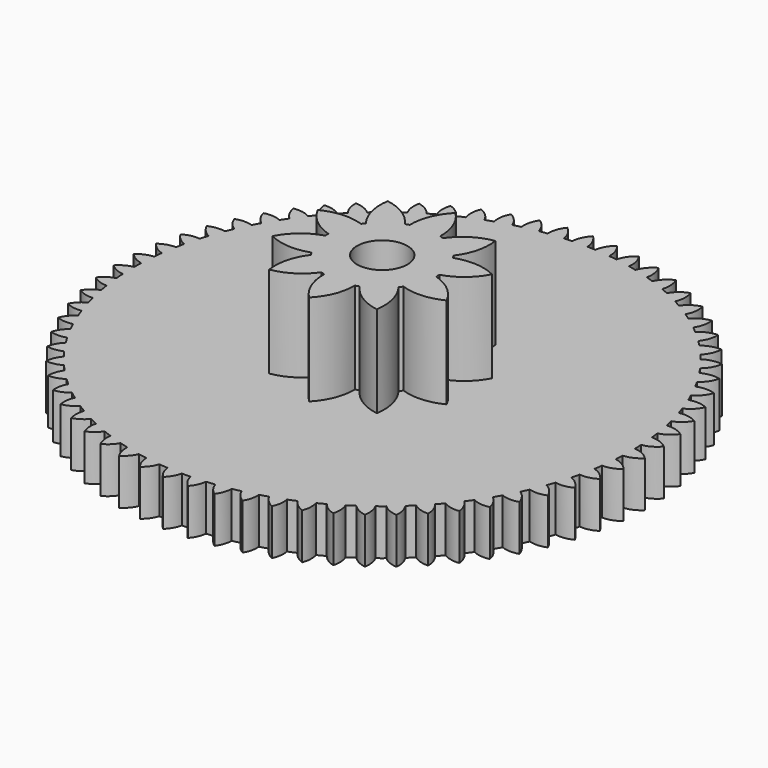
from build123d import *

# Parameters (mm, degrees)
F0_R     = 1.65
F1_DEPTH = 3
F2_R     = 1.65
F3_DEPTH = 6


# Not quite as in the source:
# - ends of sketch curves that miss each other by under 0.0002 mm in the source are joined


with BuildPart() as f1:
    # F0 (on Top) → F1 (new body)
    with BuildSketch(Plane.XY):
        with BuildLine():
            ThreePointArc((9.0030000822, 13.5880826286), (9.1966564399, 14.1755106046), (9.1611494678, 14.7930166101))
            ThreePointArc((9.1611494678, 14.7930166101), (8.5914009501, 14.5506518569), (8.1505703153, 14.1158847946))
            ThreePointArc((8.1505703153, 14.1158847946), (8.5808442549, 13.8585393124), (9.0030000822, 13.5880826286))
        make_face()
        with BuildLine():
            ThreePointArc((9.4289446926, 13.2960521202), (9.217129027, 13.4437544049), (9.0030000822, 13.5880826286))
            ThreePointArc((9.0030000822, 13.5880826286), (8.5808442549, 13.8585393124), (8.1505703153, 14.1158847946))
            ThreePointArc((8.1505703153, 14.1158847946), (7.9259223043, 14.2432354339), (7.6992849845, 14.3670111967))
            ThreePointArc((7.6992849845, 14.3670111967), (7.2538096086, 14.5969944222), (6.8014721873, 14.8131690089))
            ThreePointArc((6.8014721873, 14.8131690089), (6.5658701311, 14.9190934517), (6.3286190498, 15.021270949))
            ThreePointArc((6.3286190498, 15.021270949), (5.8637320087, 15.2087687513), (5.3932993637, 15.3818829138))
            ThreePointArc((5.3932993637, 15.3818829138), (5.1487014639, 15.4654735859), (4.9028087723, 15.5451750116))
            ThreePointArc((4.9028087723, 15.5451750116), (4.4225920082, 15.6885525122), (3.9381944266, 15.8170991227))
            ThreePointArc((3.9381944266, 15.8170991227), (3.6866298432, 15.8776182219), (3.4341363204, 15.9341365544))
            ThreePointArc((3.4341363204, 15.9341365544), (2.9428106044, 16.0321510019), (2.4487046995, 16.1150192459))
            ThreePointArc((2.4487046995, 16.1150192459), (2.1922594094, 16.1519038717), (1.9352602606, 16.1847078356))
            ThreePointArc((1.9352602606, 16.1847078356), (1.4371485303, 16.2365206895), (0.9376801939, 16.2730069703))
            ThreePointArc((0.9376801939, 16.2730069703), (0.6784826729, 16.285873058), (0.4191131655, 16.294610893))
            ThreePointArc((0.4191131655, 16.294610893), (-0.0813974371, 16.2997967612), (-0.5818312843, 16.2896124066))
            ThreePointArc((-0.5818312843, 16.2896124066), (-0.8416244022, 16.2782575347), (-1.1012033162, 16.2627596445))
            ThreePointArc((-1.1012033162, 16.2627596445), (-1.5997005284, 16.2213118526), (-2.0966911996, 16.1645874062))
            ThreePointArc((-2.0966911996, 16.1645874062), (-2.3549093713, 16.1289925864), (-2.6125253335, 16.0892731776))
            ThreePointArc((-2.6125253335, 16.0892731776), (-3.1046117426, 16.0016057297), (-3.5937788116, 15.898891592))
            ThreePointArc((-3.5937788116, 15.898891592), (-3.8482516748, 15.8392221731), (-4.1017350369, 15.7754800145))
            ThreePointArc((-4.1017350369, 15.7754800145), (-4.5830686305, 15.6424257047), (-5.0601004033, 15.4946888936))
            ThreePointArc((-5.0601004033, 15.4946888936), (-5.3086716945, 15.4112947165), (-5.5558694671, 15.3239131577))
            ThreePointArc((-5.5558694671, 15.3239131577), (-6.0222043805, 15.1467176114), (-6.4828984155, 14.9553344374))
            ThreePointArc((-6.4828984155, 14.9553344374), (-6.7234397626, 14.8487493668), (-6.9622294443, 14.7382957347))
            ThreePointArc((-6.9622294443, 14.7382957347), (-7.4094564492, 14.5186072034), (-7.849759659, 14.2853517036))
            ThreePointArc((-7.849759659, 14.2853517036), (-8.0801843427, 14.1562926286), (-8.30848773, 14.0235170924))
            ThreePointArc((-8.30848773, 14.0235170924), (-8.7326739373, 13.7633718944), (-9.1487217401, 13.4903999393))
            ThreePointArc((-9.1487217401, 13.4903999393), (-9.3669985632, 13.3397652872), (-9.58279568, 13.1855992263))
            ThreePointArc((-9.58279568, 13.1855992263), (-9.9802228808, 12.8874028124), (-10.3683768216, 12.5772318928))
            ThreePointArc((-10.3683768216, 12.5772318928), (-10.5725442468, 12.4060996349), (-10.7738875549, 12.2316534841))
            ThreePointArc((-10.7738875549, 12.2316534841), (-11.1410885881, 11.8981572133), (-11.4979718234, 11.553642021))
            ThreePointArc((-11.4979718234, 11.553642021), (-11.6861525459, 11.3632670774), (-11.8711816007, 11.1698275459))
            ThreePointArc((-11.8711816007, 11.1698275459), (-12.2049741298, 10.8041013736), (-12.5275041682, 10.4284054062))
            ThreePointArc((-12.5275041682, 10.4284054062), (-12.6979202699, 10.2202162805), (-12.8648769609, 10.0092427676))
            ThreePointArc((-12.8648769609, 10.0092427676), (-13.1623940629, 9.6146441709), (-13.4478121818, 9.2112077125))
            ThreePointArc((-13.4478121818, 9.2112077125), (-13.5988009688, 8.9868021127), (-13.7460454412, 8.7599220731))
            ThreePointArc((-13.7460454412, 8.7599220731), (-14.0047624615, 8.3400616543), (-14.2506592775, 7.9125665972))
            ThreePointArc((-14.2506592775, 7.9125665972), (-14.3806898368, 7.6737057422), (-14.5067171174, 7.4327086904))
            ThreePointArc((-14.5067171174, 7.4327086904), (-14.7244743242, 6.99141301), (-14.9288110791, 6.543745087))
            ThreePointArc((-14.9288110791, 6.543745087), (-15.0365015014, 6.2923463509), (-15.1399587627, 6.0391761578))
            ThreePointArc((-15.1399587627, 6.0391761578), (-15.3149794404, 5.5804484355), (-15.4761046744, 5.116657513))
            ThreePointArc((-15.4761046744, 5.116657513), (-15.5602397855, 4.8547850434), (-15.6399440785, 4.5915301613))
            ThreePointArc((-15.6399440785, 4.5915301613), (-15.770847824, 4.1195095475), (-15.8875092367, 3.6437686881))
            ThreePointArc((-15.8875092367, 3.6437686881), (-15.9470585693, 3.3736216428), (-16.002014739, 3.1025029077))
            ThreePointArc((-16.002014739, 3.1025029077), (-16.0878258672, 2.6214230612), (-16.1591773062, 2.1379870876))
            ThreePointArc((-16.1591773062, 2.1379870876), (-16.1933129281, 1.8618851773), (-16.2227313155, 1.5852408858))
            ThreePointArc((-16.2227313155, 1.5852408858), (-16.2628824235, 1.0993885941), (-16.2884860859, 0.6125528792))
            ThreePointArc((-16.2884860859, 0.6125528792), (-16.2965997973, 0.332918977), (-16.299913225, 0.053187011))
            ThreePointArc((-16.299913225, 0.053187011), (-16.294244109, -0.4331384488), (-16.2740681794, -0.9190782843))
            ThreePointArc((-16.2740681794, -0.9190782843), (-16.2557875013, -1.1997386011), (-16.2326669563, -1.4800417175))
            ThreePointArc((-16.2326669563, -1.4800417175), (-16.1814192039, -1.9625678452), (-16.1158312757, -2.4433547209))
            ThreePointArc((-16.1158312757, -2.4433547209), (-16.0710335889, -2.7224767002), (-16.0214019554, -3.0007797959))
            ThreePointArc((-16.0214019554, -3.0007797959), (-15.9252096446, -3.4752982285), (-15.8149663764, -3.9467503738))
            ThreePointArc((-15.8149663764, -3.9467503738), (-15.7437905398, -4.2217365432), (-15.6678337086, -4.4954406771))
            ThreePointArc((-15.6678337086, -4.4954406771), (-15.5277107264, -4.9578422318), (-15.3739442553, -5.4158875575))
            ThreePointArc((-15.3739442553, -5.4158875575), (-15.276799039, -5.6841367966), (-15.1749737341, -5.9506446852))
            ThreePointArc((-15.1749737341, -5.9506446852), (-14.9922982747, -6.3969518086), (-14.7964999486, -6.8376596341))
            ThreePointArc((-14.7964999486, -6.8376596341), (-14.6740686653, -7.0965983968), (-14.5471063814, -7.3533459001))
            ThreePointArc((-14.5471063814, -7.3533459001), (-14.3236031916, -7.7797423872), (-14.0876051855, -8.1993524218))
            ThreePointArc((-14.0876051855, -8.1993524218), (-13.9408459922, -8.4464674878), (-13.7897525324, -8.6909565121))
            ThreePointArc((-13.7897525324, -8.6909565121), (-13.5274734488, -9.0938144962), (-13.2534287945, -9.4887631011))
            ThreePointArc((-13.2534287945, -9.4887631011), (-13.0835702639, -9.7216351068), (-12.9096204994, -9.9514671563))
            ThreePointArc((-12.9096204994, -9.9514671563), (-12.6109237593, -10.3273714922), (-12.3012852517, -10.6943153664))
            ThreePointArc((-12.3012852517, -10.6943153664), (-12.1098169722, -10.9106522674), (-11.9145446105, -11.1235617823))
            ThreePointArc((-11.9145446105, -11.1235617823), (-11.582073327, -11.4693320401), (-11.2395716767, -11.8051695678))
            ThreePointArc((-11.2395716767, -11.8051695678), (-11.0282298241, -12.0028391203), (-10.8134121581, -12.1967256876))
            ThreePointArc((-10.8134121581, -12.1967256876), (-10.4500722423, -12.5094360437), (-10.0776937294, -12.811326594))
            ThreePointArc((-10.0776937294, -12.811326594), (-9.8484417487, -12.988386933), (-9.6160795585, -13.161345445))
            ThreePointArc((-9.6160795585, -13.161345445), (-9.225017246, -13.4383427852), (-8.8259810083, -13.7037242836))
            ThreePointArc((-8.8259810083, -13.7037242836), (-8.5809857451, -13.8584517044), (-8.333278722, -14.0087995825))
            ThreePointArc((-8.333278722, -14.0087995825), (-7.9178577402, -14.2477201266), (-7.4955927057, -14.4743251998))
            ThreePointArc((-7.4955927057, -14.4743251998), (-7.237196513, -14.6052383285), (-6.9765147608, -14.7315390164))
            ThreePointArc((-6.9765147608, -14.7315390164), (-6.5402930578, -14.9303237312), (-6.0984144225, -15.1161946776))
            ThreePointArc((-6.0984144225, -15.1161946776), (-5.8291039358, -15.222074343), (-5.5579562658, -15.3231564029))
            ThreePointArc((-5.5579562658, -15.3231564029), (-5.1046621281, -15.4800653926), (-4.6469471904, -15.6235681523))
            ThreePointArc((-4.6469471904, -15.6235681523), (-4.3693195954, -15.7034724272), (-4.0903194566, -15.7784437364))
            ThreePointArc((-4.0903194566, -15.7784437364), (-3.623826778, -15.8920697042), (-3.1541898812, -15.9919068967))
            ThreePointArc((-3.1541898812, -15.9919068967), (-2.8709175899, -16.0451809648), (-2.586747562, -16.0934377014))
            ThreePointArc((-2.586747562, -16.0934377014), (-2.1110499912, -16.1627184574), (-1.6335163018, -16.2179414382))
            ThreePointArc((-1.6335163018, -16.2179414382), (-1.3473109969, -16.2442221444), (-1.0606868072, -16.2654524529))
            ThreePointArc((-1.0606868072, -16.2654524529), (-0.5798705096, -16.2896823232), (-0.0985483692, -16.2997020899))
            ThreePointArc((-0.0985483692, -16.2997020899), (0.1878746276, -16.2989172378), (0.4742396132, -16.2930996679))
            ThreePointArc((0.4742396132, -16.2930996679), (0.9560248047, -16.2719395455), (1.4369731652, -16.2365362107))
            ThreePointArc((1.4369731652, -16.2365362107), (1.7209292981, -16.208898863), (2.0043582192, -16.1762958717))
            ThreePointArc((2.0043582192, -16.1762958717), (2.4829294146, -16.1097815479), (2.9593189276, -16.0291119992))
            ThreePointArc((2.9593189276, -16.0291119992), (3.2381867777, -15.9751102153), (3.5160712707, -15.9162571863))
            ThreePointArc((3.5160712707, -15.9162571863), (3.9872449379, -15.8048055289), (4.4549005417, -15.679408827))
            ThreePointArc((4.4549005417, -15.679408827), (4.7261514878, -15.5997914125), (4.9959808706, -15.5154817889))
            ThreePointArc((4.9959808706, -15.5154817889), (5.4556069796, -15.3598942862), (5.9103981417, -15.1906943161))
            ThreePointArc((5.9103981417, -15.1906943161), (6.1716227917, -15.086453265), (6.4310099498, -14.9777204883))
            ThreePointArc((6.4310099498, -14.9777204883), (6.8750076331, -14.7791836732), (7.3128843159, -14.5674885612))
            ThreePointArc((7.3128843159, -14.5674885612), (7.5618153624, -14.4398389335), (7.8085190163, -14.3079359368))
            ThreePointArc((7.8085190163, -14.3079359368), (8.2329134007, -14.0680182306), (8.649943091, -13.8155160788))
            ThreePointArc((8.649943091, -13.8155160788), (8.8844744205, -13.6658740764), (9.1164176299, -13.5122510929))
            ThreePointArc((9.1164176299, -13.5122510929), (9.5173773706, -13.2328956765), (9.9097826779, -12.9416462352))
            ThreePointArc((9.9097826779, -12.9416462352), (10.127984731, -12.7716062141), (10.3432696568, -12.5978876327))
            ThreePointArc((10.3432696568, -12.5978876327), (10.7171445996, -12.2814010451), (11.0813408248, -11.9538230506))
            ThreePointArc((11.0813408248, -11.9538230506), (11.2814723554, -11.7651341468), (11.4783914485, -11.5730950811))
            ThreePointArc((11.4783914485, -11.5730950811), (11.821749768, -11.2221313672), (12.1543817722, -10.8609853943))
            ThreePointArc((12.1543817722, -10.8609853943), (12.3348982791, -10.6555283512), (12.5119421839, -10.4470714934))
            ThreePointArc((12.5119421839, -10.4470714934), (12.8216062992, -10.0646118608), (13.1195839644, -9.672978683))
            ThreePointArc((13.1195839644, -9.672978683), (13.2791431614, -9.4527433531), (13.4350057127, -9.2298765701))
            ThreePointArc((13.4350057127, -9.2298765701), (13.7080862704, -8.8192046583), (13.9686178379, -8.4004592553))
            ThreePointArc((13.9686178379, -8.4004592553), (14.1060825888, -8.1675231251), (14.239663333, -7.9323381272))
            ThreePointArc((14.239663333, -7.9323381272), (14.4735905711, -7.4970111364), (14.6942131786, -7.0547926307))
            ThreePointArc((14.6942131786, -7.0547926307), (14.8086523452, -6.8113005893), (14.9190570363, -6.5659528743))
            ThreePointArc((14.9190570363, -6.5659528743), (15.1116089004, -6.1097689352), (15.2902156993, -5.6479468719))
            ThreePointArc((15.2902156993, -5.6479468719), (15.3809033434, -5.3960923213), (15.4674428522, -5.1427824777))
            ThreePointArc((15.4674428522, -5.1427824777), (15.6167693178, -4.6697447547), (15.7516326483, -4.1923822479))
            ThreePointArc((15.7516326483, -4.1923822479), (15.8180459886, -3.9343895465), (15.8802340211, -3.6753458931))
            ThreePointArc((15.8802340211, -3.6753458931), (15.9848771873, -3.1896240073), (16.0746673984, -2.7009383613))
            ThreePointArc((16.0746673984, -2.7009383613), (16.1164838644, -2.4390465037), (16.1540338229, -2.1765089587))
            ThreePointArc((16.1540338229, -2.1765089587), (16.2129434621, -1.6823983754), (16.2567430936, -1.1867198442))
            ThreePointArc((16.2567430936, -1.1867198442), (16.2738367414, -0.9231672187), (16.2866579831, -0.6593722322))
            ThreePointArc((16.2866579831, -0.6593722322), (16.2966641544, -0.3297536012), (16.3, 0))
            ThreePointArc((16.3, 0), (16.2991288609, 0.1685181762), (16.2965155367, 0.3370183397))
            ThreePointArc((16.2965155367, 0.3370183397), (16.2889530058, 0.6000083117), (16.277146671, 0.862841962))
            ThreePointArc((16.277146671, 0.862841962), (16.2431185974, 1.3605507092), (16.1938755894, 1.8569850281))
            ThreePointArc((16.1938755894, 1.8569850281), (16.161911698, 2.1172175764), (16.1257661929, 2.3769023314))
            ThreePointArc((16.1257661929, 2.3769023314), (16.0453843252, 2.8697808032), (15.9499414264, 3.3599655496))
            ThreePointArc((15.9499414264, 3.3599655496), (15.8940144224, 3.6152877536), (15.8340005672, 3.8696803533))
            ThreePointArc((15.8340005672, 3.8696803533), (15.7079061927, 4.3533530803), (15.567041036, 4.8329321726))
            ThreePointArc((15.567041036, 4.8329321726), (15.4877674568, 5.0812458318), (15.4045332451, 5.3282600819))
            ThreePointArc((15.4045332451, 5.3282600819), (15.2337827514, 5.7984362619), (15.0486853948, 6.263151594))
            ThreePointArc((15.0486853948, 6.263151594), (14.9468544415, 6.5024258785), (14.84121931, 6.7400452069))
            ThreePointArc((14.84121931, 6.7400452069), (14.6272726747, 7.1925582445), (14.3995327667, 7.6382888203))
            ThreePointArc((14.3995327667, 7.6382888203), (14.2761000685, 7.8665727502), (14.1490485526, 8.0928625996))
            ThreePointArc((14.1490485526, 8.0928625996), (13.8937541972, 8.5237077793), (13.6253445867, 8.9465068543))
            ThreePointArc((13.6253445867, 8.9465068543), (13.4814252261, 9.1619415995), (13.334099868, 9.3750616377))
            ThreePointArc((13.334099868, 9.3750616377), (13.0396762367, 9.7804316695), (12.7329333954, 10.1765616565))
            ThreePointArc((12.7329333954, 10.1765616565), (12.5697940741, 10.3773925884), (12.4034874665, 10.5756086665))
            ThreePointArc((12.4034874665, 10.5756086665), (12.0725016783, 10.9519269185), (11.730103288, 11.3178918909))
            ThreePointArc((11.730103288, 11.3178918909), (11.549153545, 11.5024802714), (11.3652994227, 11.68417601))
            ThreePointArc((11.3652994227, 11.68417601), (11.0006433175, 12.0281273107), (10.6255833433, 12.3607029984))
            ThreePointArc((10.6255833433, 12.3607029984), (10.4283657755, 12.5275371583), (10.2285291094, 12.6912250101))
            ThreePointArc((10.2285291094, 12.6912250101), (9.8333929684, 12.9997839493), (9.4289446926, 13.2960521202))
        make_face()
        Circle(F0_R, mode=Mode.SUBTRACT)
        with BuildLine():
            ThreePointArc((-13.4478121818, 9.2112077125), (-13.1623940629, 9.6146441709), (-12.8648769609, 10.0092427676))
            ThreePointArc((-12.8648769609, 10.0092427676), (-13.4046707125, 10.205028848), (-13.9788739128, 10.2046185496))
            ThreePointArc((-13.9788739128, 10.2046185496), (-13.8004482307, 9.6613480768), (-13.4478121818, 9.2112077125))
        make_face()
        with BuildLine():
            ThreePointArc((-14.7964999486, -6.8376596341), (-14.9922982747, -6.3969518086), (-15.1749737341, -5.9506446852))
            ThreePointArc((-15.1749737341, -5.9506446852), (-15.5708692449, -6.3015074646), (-15.8358560483, -6.7593501663))
            ThreePointArc((-15.8358560483, -6.7593501663), (-15.3225027363, -6.8824494732), (-14.7964999486, -6.8376596341))
        make_face()
        with BuildLine():
            ThreePointArc((-15.8875092367, 3.6437686881), (-15.770847824, 4.1195095475), (-15.6399440785, 4.5915301613))
            ThreePointArc((-15.6399440785, 4.5915301613), (-16.195084245, 4.5669767558), (-16.710815914, 4.3600847069))
            ThreePointArc((-16.710815914, 4.3600847069), (-16.3598933634, 3.932125015), (-15.8875092367, 3.6437686881))
        make_face()
        with BuildLine():
            ThreePointArc((-10.0776937294, -12.811326594), (-10.4500722423, -12.5094360437), (-10.8134121581, -12.1967256876))
            ThreePointArc((-10.8134121581, -12.1967256876), (-11.0005101632, -12.6816290806), (-11.0280129906, -13.2006479227))
            ThreePointArc((-11.0280129906, -13.2006479227), (-10.5218960294, -13.0815529808), (-10.0776937294, -12.811326594))
        make_face()
        with BuildLine():
            ThreePointArc((-12.5275041682, 10.4284054062), (-12.2049741298, 10.8041013736), (-11.8711816007, 11.1698275459))
            ThreePointArc((-11.8711816007, 11.1698275459), (-12.3933786753, 11.419483248), (-12.9696046122, 11.4740856662))
            ThreePointArc((-12.9696046122, 11.4740856662), (-12.8410090509, 10.9121568701), (-12.5275041682, 10.4284054062))
        make_face()
        with BuildLine():
            ThreePointArc((-9.1487217401, 13.4903999393), (-8.7326739373, 13.7633718944), (-8.30848773, 14.0235170924))
            ThreePointArc((-8.30848773, 14.0235170924), (-8.7458498526, 14.4223622655), (-9.2955761569, 14.6418254487))
            ThreePointArc((-9.2955761569, 14.6418254487), (-9.3263886042, 14.0528178228), (-9.1487217401, 13.4903999393))
        make_face()
        with BuildLine():
            ThreePointArc((-15.8149663764, -3.9467503738), (-15.9252096446, -3.4752982285), (-16.0214019554, -3.0007797959))
            ThreePointArc((-16.0214019554, -3.0007797959), (-16.482789605, -3.2722344372), (-16.833413186, -3.6767456113))
            ThreePointArc((-16.833413186, -3.6767456113), (-16.3462469014, -3.8949465389), (-15.8149663764, -3.9467503738))
        make_face()
        with BuildLine():
            ThreePointArc((-11.4979718234, 11.553642021), (-11.1410885881, 11.8981572133), (-10.7738875549, 12.2316534841))
            ThreePointArc((-10.7738875549, 12.2316534841), (-11.2730333724, 12.5335063603), (-11.8458952673, 12.6434652408))
            ThreePointArc((-11.8458952673, 12.6434652408), (-11.7690792198, 12.0675401078), (-11.4979718234, 11.553642021))
        make_face()
        with BuildLine():
            ThreePointArc((-6.9037466713, -15.7547598521), (-6.4502625987, -15.4995667802), (-6.0984144225, -15.1161946776))
            ThreePointArc((-6.0984144225, -15.1161946776), (-6.5402930578, -14.9303237312), (-6.9765147608, -14.7315390164))
            ThreePointArc((-6.9765147608, -14.7315390164), (-7.0213957965, -15.2489287386), (-6.9037466713, -15.7547598521))
        make_face()
        with BuildLine():
            ThreePointArc((-15.4761046744, 5.116657513), (-15.3149794404, 5.5804484355), (-15.1399587627, 6.0391761578))
            ThreePointArc((-15.1399587627, 6.0391761578), (-15.6993958255, 6.0692886235), (-16.2368332658, 5.9110559285))
            ThreePointArc((-16.2368332658, 5.9110559285), (-15.9243820333, 5.4488220885), (-15.4761046744, 5.116657513))
        make_face()
        with BuildLine():
            ThreePointArc((-15.3739442553, -5.4158875575), (-15.5277107264, -4.9578422318), (-15.6678337086, -4.4954406771))
            ThreePointArc((-15.6678337086, -4.4954406771), (-16.0981273864, -4.808275934), (-16.4069584338, -5.241452493))
            ThreePointArc((-16.4069584338, -5.241452493), (-15.9046157812, -5.4125526093), (-15.3739442553, -5.4158875575))
        make_face()
        with BuildLine():
            ThreePointArc((-14.0876051855, -8.1993524218), (-14.3236031916, -7.7797423872), (-14.5471063814, -7.3533459001))
            ThreePointArc((-14.5471063814, -7.3533459001), (-14.905666898, -7.738679317), (-15.1251248979, -8.2170992919))
            ThreePointArc((-15.1251248979, -8.2170992919), (-14.6049384056, -8.2916300343), (-14.0876051855, -8.1993524218))
        make_face()
        with BuildLine():
            ThreePointArc((-14.2506592775, 7.9125665972), (-14.0047624615, 8.3400616543), (-13.7460454412, 8.7599220731))
            ThreePointArc((-13.7460454412, 8.7599220731), (-14.2979036878, 8.9007679602), (-14.8648336743, 8.8462200137))
            ThreePointArc((-14.8648336743, 8.8462200137), (-14.6389245816, 8.3259928538), (-14.2506592775, 7.9125665972))
        make_face()
        with BuildLine():
            ThreePointArc((-7.849759659, 14.2853517036), (-7.4094564492, 14.5186072034), (-6.9622294443, 14.7382957347))
            ThreePointArc((-6.9622294443, 14.7382957347), (-7.3613861749, 15.1807873454), (-7.8913786874, 15.4532444206))
            ThreePointArc((-7.8913786874, 15.4532444206), (-7.9770667207, 14.8655029152), (-7.849759659, 14.2853517036))
        make_face()
        with BuildLine():
            ThreePointArc((-12.3012852517, -10.6943153664), (-12.6109237593, -10.3273714922), (-12.9096204994, -9.9514671563))
            ThreePointArc((-12.9096204994, -9.9514671563), (-13.1861628926, -10.3944543984), (-13.3109321991, -10.901550062))
            ThreePointArc((-13.3109321991, -10.901550062), (-12.7895674091, -10.8785219679), (-12.3012852517, -10.6943153664))
        make_face()
        with BuildLine():
            ThreePointArc((-14.9288110791, 6.543745087), (-14.7244743242, 6.99141301), (-14.5067171174, 7.4327086904))
            ThreePointArc((-14.5067171174, 7.4327086904), (-15.065102191, 7.5181378295), (-15.6196980504, 7.4108277136))
            ThreePointArc((-15.6196980504, 7.4108277136), (-15.3490088627, 6.9177225607), (-14.9288110791, 6.543745087))
        make_face()
        with BuildLine():
            ThreePointArc((-8.3564404679, -15.0337522137), (-7.8815477586, -14.8224674568), (-7.4955927057, -14.4743251998))
            ThreePointArc((-7.4955927057, -14.4743251998), (-7.9178577402, -14.2477201266), (-8.333278722, -14.0087995825))
            ThreePointArc((-8.333278722, -14.0087995825), (-8.4262129098, -14.5194374865), (-8.3564404679, -15.0337522137))
        make_face()
        with BuildLine():
            ThreePointArc((-16.1158312757, -2.4433547209), (-16.1814192039, -1.9625678452), (-16.2326669563, -1.4800417175))
            ThreePointArc((-16.2326669563, -1.4800417175), (-16.7214817518, -1.707010172), (-17.1114726052, -2.0789802216))
            ThreePointArc((-17.1114726052, -2.0789802216), (-16.643614818, -2.343040048), (-16.1158312757, -2.4433547209))
        make_face()
        with BuildLine():
            ThreePointArc((-16.1591773062, 2.1379870876), (-16.0878258672, 2.6214230612), (-16.002014739, 3.1025029077))
            ThreePointArc((-16.002014739, 3.1025029077), (-16.5476918541, 3.0244519816), (-17.0374806185, 2.7715440394))
            ThreePointArc((-17.0374806185, 2.7715440394), (-16.6516088073, 2.3809034361), (-16.1591773062, 2.1379870876))
        make_face()
        with BuildLine():
            ThreePointArc((-6.4828984155, 14.9553344374), (-6.0222043805, 15.1467176114), (-5.5558694671, 15.3239131577))
            ThreePointArc((-5.5558694671, 15.3239131577), (-5.9124159248, 15.806102838), (-6.4173688056, 16.1296068603))
            ThreePointArc((-6.4173688056, 16.1296068603), (-6.557944508, 15.5484869751), (-6.4828984155, 14.9553344374))
        make_face()
        with BuildLine():
            ThreePointArc((-11.2395716767, -11.8051695678), (-11.582073327, -11.4693320401), (-11.9145446105, -11.1235617823))
            ThreePointArc((-11.9145446105, -11.1235617823), (-12.1471198445, -11.5895110151), (-12.2234138413, -12.1046606566))
            ThreePointArc((-12.2234138413, -12.1046606566), (-11.7076432212, -12.0332619538), (-11.2395716767, -11.8051695678))
        make_face()
        with BuildLine():
            ThreePointArc((-16.2884860859, 0.6125528792), (-16.2628824235, 1.0993885941), (-16.2227313155, 1.5852408858))
            ThreePointArc((-16.2227313155, 1.5852408858), (-16.7540115164, 1.4553392821), (-17.2139566382, 1.1593940787))
            ThreePointArc((-17.2139566382, 1.1593940787), (-16.7968491197, 0.8087533534), (-16.2884860859, 0.6125528792))
        make_face()
        with BuildLine():
            ThreePointArc((-16.2740681794, -0.9190782843), (-16.294244109, -0.4331384488), (-16.299913225, 0.053187011))
            ThreePointArc((-16.299913225, 0.053187011), (-16.8121367183, -0.1264833663), (-17.2386930954, -0.4621975435))
            ThreePointArc((-17.2386930954, -0.4621975435), (-16.7942172736, -0.770523448), (-16.2740681794, -0.9190782843))
        make_face()
        with BuildLine():
            ThreePointArc((-8.8259810083, -13.7037242836), (-9.225017246, -13.4383427852), (-9.6160795585, -13.161345445))
            ThreePointArc((-9.6160795585, -13.161345445), (-9.7565232482, -13.661152592), (-9.7352348726, -14.1798802848))
            ThreePointArc((-9.7352348726, -14.1798802848), (-9.2427687159, -14.0140589838), (-8.8259810083, -13.7037242836))
        make_face()
        with BuildLine():
            ThreePointArc((-13.2534287945, -9.4887631011), (-13.5274734488, -9.0938144962), (-13.7897525324, -8.6909565121))
            ThreePointArc((-13.7897525324, -8.6909565121), (-14.1084080205, -9.10704034), (-14.2810109135, -9.6018891181))
            ThreePointArc((-14.2810109135, -9.6018891181), (-13.7581616829, -9.6276061629), (-13.2534287945, -9.4887631011))
        make_face()
        with BuildLine():
            ThreePointArc((5.7635119098, -16.2452018746), (5.924054002, -15.7300804318), (5.9103981417, -15.1906943161))
            ThreePointArc((5.9103981417, -15.1906943161), (5.4556069796, -15.3598942862), (4.9959808706, -15.5154817889))
            ThreePointArc((4.9959808706, -15.5154817889), (5.3198105511, -15.943383288), (5.7635119098, -16.2452018746))
        make_face()
        with BuildLine():
            ThreePointArc((8.7082914796, -14.8939637866), (8.7695504309, -14.3498471333), (8.649943091, -13.8155160788))
            ThreePointArc((8.649943091, -13.8155160788), (8.2329134007, -14.0680182306), (7.8085190163, -14.3079359368))
            ThreePointArc((7.8085190163, -14.3079359368), (8.2095640216, -14.6759394559), (8.7082914796, -14.8939637866))
        make_face()
        with BuildLine():
            ThreePointArc((13.5944237096, -10.6811506211), (13.44439849, -10.1359025713), (13.1195839644, -9.672978683))
            ThreePointArc((13.1195839644, -9.672978683), (12.8216062992, -10.0646118608), (12.5119421839, -10.4470714934))
            ThreePointArc((12.5119421839, -10.4470714934), (13.0330247895, -10.657330957), (13.5944237096, -10.6811506211))
        make_face()
        with BuildLine():
            ThreePointArc((-3.8282634433, -16.7740605928), (-3.4286781395, -16.4368891419), (-3.1541898812, -15.9919068967))
            ThreePointArc((-3.1541898812, -15.9919068967), (-3.623826778, -15.8920697042), (-4.0903194566, -15.7784437364))
            ThreePointArc((-4.0903194566, -15.7784437364), (-4.038666053, -16.29714433), (-3.8282634433, -16.7740605928))
        make_face()
        with BuildLine():
            ThreePointArc((12.5267609096, -11.90191572), (12.4300439072, -11.349442923), (12.1543817722, -10.8609853943))
            ThreePointArc((12.1543817722, -10.8609853943), (11.821749768, -11.2221313672), (11.4783914485, -11.5730950811))
            ThreePointArc((11.4783914485, -11.5730950811), (11.9744970624, -11.8270292467), (12.5267609096, -11.90191572))
        make_face()
        with BuildLine():
            ThreePointArc((16.5973095343, -4.9710928578), (16.2442453802, -4.5059629293), (15.7516326483, -4.1923822479))
            ThreePointArc((15.7516326483, -4.1923822479), (15.6167693178, -4.6697447547), (15.4674428522, -5.1427824777))
            ThreePointArc((15.4674428522, -5.1427824777), (16.0476636589, -5.157542457), (16.5973095343, -4.9710928578))
        make_face()
        with BuildLine():
            ThreePointArc((-0.6166574992, -17.2020306208), (-0.2848584764, -16.7926355851), (-0.0985483692, -16.2997020899))
            ThreePointArc((-0.0985483692, -16.2997020899), (-0.5798705096, -16.2896823232), (-1.0606868072, -16.2654524529))
            ThreePointArc((-1.0606868072, -16.2654524529), (-0.9138726474, -16.7693938984), (-0.6166574992, -17.2020306208))
        make_face()
        with BuildLine():
            ThreePointArc((15.3643957007, -7.967339604), (15.1097540709, -7.4519832007), (14.6942131786, -7.0547926307))
            ThreePointArc((14.6942131786, -7.0547926307), (14.4735905711, -7.4970111364), (14.239663333, -7.9323381272))
            ThreePointArc((14.239663333, -7.9323381272), (14.7989638858, -8.0483494079), (15.3643957007, -7.967339604))
        make_face()
        with BuildLine():
            ThreePointArc((10.0729125407, -14.0176187399), (10.0823022102, -13.4658427192), (9.9097826779, -12.9416462352))
            ThreePointArc((9.9097826779, -12.9416462352), (9.5173773706, -13.2328956765), (9.1164176299, -13.5122510929))
            ThreePointArc((9.1164176299, -13.5122510929), (9.5522140686, -13.8452807431), (10.0729125407, -14.0176187399))
        make_face()
        with BuildLine():
            ThreePointArc((1.0050683717, -17.1887459991), (1.2981820658, -16.7476400459), (1.4369731652, -16.2365362107))
            ThreePointArc((1.4369731652, -16.2365362107), (0.9560248047, -16.2719395455), (0.4742396132, -16.2930996679))
            ThreePointArc((0.4742396132, -16.2930996679), (0.6674016185, -16.7837451359), (1.0050683717, -17.1887459991))
        make_face()
        with BuildLine():
            ThreePointArc((14.5430809179, -9.365772051), (14.3402403265, -8.8328941245), (13.9686178379, -8.4004592553))
            ThreePointArc((13.9686178379, -8.4004592553), (13.7080862704, -8.8192046583), (13.4350057127, -9.2298765701))
            ThreePointArc((13.4350057127, -9.2298765701), (13.9772408237, -9.3940603895), (14.5430809179, -9.365772051))
        make_face()
        with BuildLine():
            ThreePointArc((-5.3899198082, -16.3365669591), (-4.9615776742, -16.0393135471), (-4.6469471904, -15.6235681523))
            ThreePointArc((-4.6469471904, -15.6235681523), (-5.1046621281, -15.4800653926), (-5.5579562658, -15.3231564029))
            ThreePointArc((-5.5579562658, -15.3231564029), (-5.5545430133, -15.8432270191), (-5.3899198082, -16.3365669591))
        make_face()
        with BuildLine():
            ThreePointArc((11.3494751768, -13.0173392202), (11.3060561299, -12.4627268732), (11.0813408248, -11.9538230506))
            ThreePointArc((11.0813408248, -11.9538230506), (10.7171445996, -12.2814010451), (10.3432696568, -12.5978876327))
            ThreePointArc((10.3432696568, -12.5978876327), (10.8108508202, -12.892824754), (11.3494751768, -13.0173392202))
        make_face()
        with BuildLine():
            ThreePointArc((2.6184243581, -17.0236589241), (2.8699321758, -16.5541700687), (2.9593189276, -16.0291119992))
            ThreePointArc((2.9593189276, -16.0291119992), (2.4829294146, -16.1097815479), (2.0043582192, -16.1762958717))
            ThreePointArc((2.0043582192, -16.1762958717), (2.2426647204, -16.6497820929), (2.6184243581, -17.0236589241))
        make_face()
        with BuildLine():
            ThreePointArc((16.0511503143, -6.4981427547), (15.746255105, -6.0054069588), (15.2902156993, -5.6479468719))
            ThreePointArc((15.2902156993, -5.6479468719), (15.1116089004, -6.1097689352), (14.9190570363, -6.5659528743))
            ThreePointArc((14.9190570363, -6.5659528743), (15.4910925564, -6.6320324781), (16.0511503143, -6.4981427547))
        make_face()
        with BuildLine():
            ThreePointArc((7.2676043325, -15.6386730087), (7.3793752062, -15.106848432), (7.3128843159, -14.5674885612))
            ThreePointArc((7.3128843159, -14.5674885612), (6.8750076331, -14.7791836732), (6.4310099498, -14.9777204883))
            ThreePointArc((6.4310099498, -14.9777204883), (6.7946335685, -15.3773993044), (7.2676043325, -15.6386730087))
        make_face()
        with BuildLine():
            ThreePointArc((-2.2325014691, -17.0633960435), (-1.8651503762, -16.6887449359), (-1.6335163018, -16.2179414382))
            ThreePointArc((-1.6335163018, -16.2179414382), (-2.1110499912, -16.1627184574), (-2.586747562, -16.0934377014))
            ThreePointArc((-2.586747562, -16.0934377014), (-2.4871982071, -16.6067481687), (-2.2325014691, -17.0633960435))
        make_face()
        with BuildLine():
            ThreePointArc((4.2092322297, -16.708220187), (4.4164572314, -16.2139660696), (4.4549005417, -15.679408827))
            ThreePointArc((4.4549005417, -15.679408827), (3.9872449379, -15.8048055289), (3.5160712707, -15.9162571863))
            ThreePointArc((3.5160712707, -15.9162571863), (3.7980306451, -16.3687979289), (4.2092322297, -16.708220187))
        make_face()
        with BuildLine():
            ThreePointArc((13.9165100112, 10.4331279602), (13.3004145283, 10.4169772414), (12.7329333954, 10.1765616565))
            ThreePointArc((12.7329333954, 10.1765616565), (13.0396762367, 9.7804316695), (13.334099868, 9.3750616377))
            ThreePointArc((13.334099868, 9.3750616377), (13.72525339, 9.8490784072), (13.9165100112, 10.4331279602))
        make_face()
        with BuildLine():
            ThreePointArc((14.8246044549, 9.0894257006), (14.2114742108, 9.1312500071), (13.6253445867, 8.9465068543))
            ThreePointArc((13.6253445867, 8.9465068543), (13.8937541972, 8.5237077793), (14.1490485526, 8.0928625996))
            ThreePointArc((14.1490485526, 8.0928625996), (14.5806461991, 8.5275451177), (14.8246044549, 9.0894257006))
        make_face()
        with BuildLine():
            ThreePointArc((16.2445044144, 6.1771318983), (15.6546566409, 6.332213494), (15.0486853948, 6.263151594))
            ThreePointArc((15.0486853948, 6.263151594), (15.2337827514, 5.7984362619), (15.4045332451, 5.3282600819))
            ThreePointArc((15.4045332451, 5.3282600819), (15.9037403627, 5.674305116), (16.2445044144, 6.1771318983))
        make_face()
        with BuildLine():
            ThreePointArc((17.2499208635, -1.79750348), (16.8088917178, -1.401767562), (16.2567430936, -1.1867198442))
            ThreePointArc((16.2567430936, -1.1867198442), (16.2129434621, -1.6823983754), (16.1540338229, -2.1765089587))
            ThreePointArc((16.1540338229, -2.1765089587), (16.7362518943, -2.0861104235), (17.2499208635, -1.79750348))
        make_face()
        with BuildLine():
            ThreePointArc((11.743863897, 12.8367044512), (11.1394547215, 12.7050549318), (10.6255833433, 12.3607029984))
            ThreePointArc((10.6255833433, 12.3607029984), (11.0006433175, 12.0281273107), (11.3652994227, 11.68417601))
            ThreePointArc((11.3652994227, 11.68417601), (11.6639705514, 12.2245098824), (11.743863897, 12.8367044512))
        make_face()
        with BuildLine():
            ThreePointArc((12.8865794696, 11.6858906516), (12.273398193, 11.6117040379), (11.730103288, 11.3178918909))
            ThreePointArc((11.730103288, 11.3178918909), (12.0725016783, 10.9519269185), (12.4034874665, 10.5756086665))
            ThreePointArc((12.4034874665, 10.5756086665), (12.7501997526, 11.0849910214), (12.8865794696, 11.6858906516))
        make_face()
        with BuildLine():
            ThreePointArc((16.998073694, -3.3996096827), (16.5994582046, -2.9668935551), (16.0746673984, -2.7009383613))
            ThreePointArc((16.0746673984, -2.7009383613), (15.9848771873, -3.1896240073), (15.8802340211, -3.6753458931))
            ThreePointArc((15.8802340211, -3.6753458931), (16.4639006754, -3.6378018427), (16.998073694, -3.3996096827))
        make_face()
        with BuildLine():
            ThreePointArc((17.3506378008, -0.1788536168), (16.8708309132, 0.1756407235), (16.2965155367, 0.3370183397))
            ThreePointArc((16.2965155367, 0.3370183397), (16.2991288609, 0.1685181762), (16.3, 0))
            ThreePointArc((16.3, 0), (16.2966641544, -0.3297536012), (16.2866579831, -0.6593722322))
            ThreePointArc((16.2866579831, -0.6593722322), (16.8624180745, -0.5160302744), (17.3506378008, -0.1788536168))
        make_face()
        with BuildLine():
            ThreePointArc((10.4984055187, 13.8754559659), (9.9085302484, 13.6875435714), (9.4289544951, 13.2960451688))
            ThreePointArc((9.4289544951, 13.2960451688), (9.8333929684, 12.9997839493), (10.2285291094, 12.6912250101))
            ThreePointArc((10.2285291094, 12.6912250101), (10.4760129813, 13.2576922643), (10.4984055187, 13.8754559659))
        make_face()
        with BuildLine():
            ThreePointArc((15.6028824343, 7.6665923765), (14.998543665, 7.7657000692), (14.3995327667, 7.6382888203))
            ThreePointArc((14.3995327667, 7.6382888203), (14.6272726747, 7.1925582445), (14.84121931, 6.7400452069))
            ThreePointArc((14.84121931, 6.7400452069), (15.3089266619, 7.1319030153), (15.6028824343, 7.6665923765))
        make_face()
        with BuildLine():
            ThreePointArc((16.7438317982, 4.6341336984), (16.173977018, 4.8432843204), (15.567041036, 4.8329321726))
            ThreePointArc((15.567041036, 4.8329321726), (15.7079061927, 4.3533530803), (15.8340005672, 3.8696803533))
            ThreePointArc((15.8340005672, 3.8696803533), (16.3598843867, 4.1674426321), (16.7438317982, 4.6341336984))
        make_face()
        with BuildLine():
            ThreePointArc((17.0964764787, 3.0511577002), (16.5518524319, 3.3119085107), (15.9499414264, 3.3599655496))
            ThreePointArc((15.9499414264, 3.3599655496), (16.0453843252, 2.8697808032), (16.1257661929, 2.3769023314))
            ThreePointArc((16.1257661929, 2.3769023314), (16.6733523233, 2.6244374631), (17.0964764787, 3.0511577002))
        make_face()
        with BuildLine():
            ThreePointArc((17.2993394018, 1.4421151539), (16.7848581789, 1.7514730042), (16.1938755894, 1.8569850281))
            ThreePointArc((16.1938755894, 1.8569850281), (16.2431185974, 1.3605507092), (16.277146671, 0.862841962))
            ThreePointArc((16.277146671, 0.862841962), (16.8413694924, 1.0587309482), (17.2993394018, 1.4421151539))
        make_face()
        with BuildLine():
            ThreePointArc((6.8014721873, 14.8131690089), (7.2538096086, 14.5969944222), (7.6992849845, 14.3670111967))
            ThreePointArc((7.6992849845, 14.3670111967), (7.8370254823, 14.9699299094), (7.7438475987, 15.5813228279))
            ThreePointArc((7.7438475987, 15.5813228279), (7.1995799332, 15.2869008227), (6.8014721873, 14.8131690089))
        make_face()
        with BuildLine():
            ThreePointArc((-3.5937788116, 15.898891592), (-3.1046117426, 16.0016057297), (-2.6125253335, 16.0892731776))
            ThreePointArc((-2.6125253335, 16.0892731776), (-2.8724410639, 16.6371352927), (-3.3122260896, 17.0546256702))
            ThreePointArc((-3.3122260896, 17.0546256702), (-3.5604096752, 16.5029245087), (-3.5937788116, 15.898891592))
        make_face()
        with BuildLine():
            ThreePointArc((3.9381944266, 15.8170991227), (4.4225920082, 15.6885525122), (4.9028087723, 15.5451750116))
            ThreePointArc((4.9028087723, 15.5451750116), (4.924846055, 16.1618020733), (4.7195215923, 16.7436581035))
            ThreePointArc((4.7195215923, 16.7436581035), (4.2410014553, 16.3544642503), (3.9381944266, 15.8170991227))
        make_face()
        with BuildLine():
            ThreePointArc((5.3932993637, 15.3818829138), (5.8637320087, 15.2087687513), (6.3286190498, 15.021270949))
            ThreePointArc((6.3286190498, 15.021270949), (6.4089461065, 15.6339771467), (6.2589552109, 16.2334469558))
            ThreePointArc((6.2589552109, 16.2334469558), (5.7452183406, 15.8899127744), (5.3932993637, 15.3818829138))
        make_face()
        with BuildLine():
            ThreePointArc((-5.0601004033, 15.4946888936), (-4.5830686305, 15.6424257047), (-4.1017350369, 15.7754800145))
            ThreePointArc((-4.1017350369, 15.7754800145), (-4.4117026644, 16.2929362781), (-4.8865001635, 16.6649688704))
            ThreePointArc((-4.8865001635, 16.6649688704), (-5.08142787, 16.0958686121), (-5.0601004033, 15.4946888936))
        make_face()
        with BuildLine():
            ThreePointArc((0.9376801939, 16.2730069703), (1.4371485303, 16.2365206895), (1.9352602606, 16.1847078356))
            ThreePointArc((1.9352602606, 16.1847078356), (1.840669454, 16.7912989479), (1.5315054751, 17.3216929828))
            ThreePointArc((1.5315054751, 17.3216929828), (1.1357617098, 16.8533137442), (0.9376801939, 16.2730069703))
        make_face()
        with BuildLine():
            ThreePointArc((-0.5818312843, 16.2896124066), (-0.0813974371, 16.2997967612), (0.4191131655, 16.294610893))
            ThreePointArc((0.4191131655, 16.294610893), (0.2674910122, 16.8873020802), (-0.0890606233, 17.384436923))
            ThreePointArc((-0.0890606233, 17.384436923), (-0.438208718, 16.8832772601), (-0.5818312843, 16.2896124066))
        make_face()
        with BuildLine():
            ThreePointArc((-2.0966911996, 16.1645874062), (-1.5997005284, 16.2213118526), (-1.1012033162, 16.2627596445))
            ThreePointArc((-1.1012033162, 16.2627596445), (-1.308140876, 16.8357995973), (-1.7083813612, 17.2951529419))
            ThreePointArc((-1.7083813612, 17.2951529419), (-2.0081591925, 16.7661479613), (-2.0966911996, 16.1645874062))
        make_face()
        with BuildLine():
            ThreePointArc((2.4487046995, 16.1150192459), (2.9428106044, 16.0321510019), (3.4341363204, 15.9341365544))
            ThreePointArc((3.4341363204, 15.9341365544), (3.397649867, 16.5487289864), (3.1390753409, 17.1074725173))
            ThreePointArc((3.1390753409, 17.1074725173), (2.7000406068, 16.6765294386), (2.4487046995, 16.1150192459))
        make_face()
        with BuildLine():
            ThreePointArc((-10.3683768216, 12.5772318928), (-9.9802228808, 12.8874028124), (-9.58279568, 13.1855992263))
            ThreePointArc((-9.58279568, 13.1855992263), (-10.0535875938, 13.5373773683), (-10.6176210763, 13.7024807237))
            ThreePointArc((-10.6176210763, 13.7024807237), (-10.5940980862, 13.1174627021), (-10.3683768216, 12.5772318928))
        make_face()
    extrude(amount=F1_DEPTH)

    # F2 (on face) → F3 (join)
    with BuildSketch(Plane.XY.offset(3)):
        with BuildLine():
            ThreePointArc((1, 3.5), (0.7557417519, 4.8522967007), (0, 6))
            ThreePointArc((0, 6), (-0.7557417519, 4.8522967007), (-1, 3.5))
            Line((-1, 3.5), (-1.2482313886, 3.4193447326))
            ThreePointArc((-1.2482313886, 3.4193447326), (-2.2407005198, 4.3698043489), (-3.5267115138, 4.8541019662))
            ThreePointArc((-3.5267115138, 4.8541019662), (-3.4635163611, 3.4813766364), (-2.8662653774, 2.243774228))
            Line((-2.8662653774, 2.243774228), (-3.0196808127, 2.0326159966))
            ThreePointArc((-3.0196808127, 2.0326159966), (-4.3812713516, 2.21819526), (-5.7063390978, 1.8541019662))
            ThreePointArc((-5.7063390978, 1.8541019662), (-4.8483454409, 0.7806890245), (-3.6377148014, 0.130502964))
            Line((-3.6377148014, 0.130502964), (-3.6377148014, -0.130502964))
            ThreePointArc((-3.6377148014, -0.130502964), (-4.8483454409, -0.7806890245), (-5.7063390978, -1.8541019662))
            ThreePointArc((-5.7063390978, -1.8541019662), (-4.3812713516, -2.21819526), (-3.0196808127, -2.0326159966))
            Line((-3.0196808127, -2.0326159966), (-2.8662653774, -2.243774228))
            ThreePointArc((-2.8662653774, -2.243774228), (-3.4635163611, -3.4813766364), (-3.5267115138, -4.8541019662))
            ThreePointArc((-3.5267115138, -4.8541019662), (-2.2407005198, -4.3698043489), (-1.2482313886, -3.4193447326))
            Line((-1.2482313886, -3.4193447326), (-1, -3.5))
            ThreePointArc((-1, -3.5), (-0.7557417519, -4.8522967007), (0, -6))
            ThreePointArc((0, -6), (0.7557417519, -4.8522967007), (1, -3.5))
            Line((1, -3.5), (1.2482313886, -3.4193447326))
            ThreePointArc((1.2482313886, -3.4193447326), (2.2407005198, -4.3698043489), (3.5267115138, -4.8541019662))
            ThreePointArc((3.5267115138, -4.8541019662), (3.4635163611, -3.4813766364), (2.8662653774, -2.243774228))
            Line((2.8662653774, -2.243774228), (3.0196808127, -2.0326159966))
            ThreePointArc((3.0196808127, -2.0326159966), (4.3812713516, -2.21819526), (5.7063390978, -1.8541019662))
            ThreePointArc((5.7063390978, -1.8541019662), (4.8483454409, -0.7806890245), (3.6377148014, -0.130502964))
            Line((3.6377148014, -0.130502964), (3.6377148014, 0.130502964))
            ThreePointArc((3.6377148014, 0.130502964), (4.8483454409, 0.7806890245), (5.7063390978, 1.8541019662))
            ThreePointArc((5.7063390978, 1.8541019662), (4.3812713516, 2.21819526), (3.0196808127, 2.0326159966))
            Line((3.0196808127, 2.0326159966), (2.8662653774, 2.243774228))
            ThreePointArc((2.8662653774, 2.243774228), (3.4635163611, 3.4813766364), (3.5267115138, 4.8541019662))
            ThreePointArc((3.5267115138, 4.8541019662), (2.2407005198, 4.3698043489), (1.2482313886, 3.4193447326))
            Line((1.2482313886, 3.4193447326), (1, 3.5))
        make_face()
        Circle(F2_R, mode=Mode.SUBTRACT)
    extrude(amount=F3_DEPTH)


solid = f1.part
